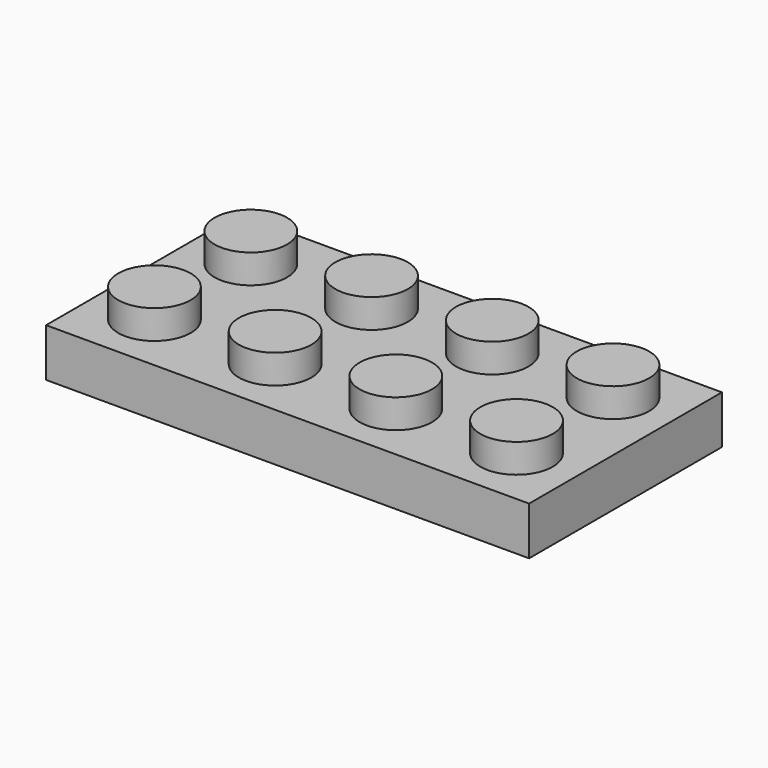
from build123d import *

# Parameters (mm, degrees)
F1_DEPTH = 3.175
F2_DEPTH = 5.08
F3_T     = -1.6002


# Not quite as in the source:
# - a feature names something its author has since deleted; it is built from what else it names


with BuildPart() as f1:
    # F0 (on Top) → F1 (new body)
    with BuildSketch(Plane.XY):
        with BuildLine():
            Line((-6.9955831819, 8.5962191019), (-38.8090831819, 8.5962191019))
            Line((-38.8090831819, 8.5962191019), (-38.8090831819, 4.6274691019))
            Line((-38.8090831819, 4.6274691019), (-37.2342831819, 4.6274691019))
            ThreePointArc((-37.2342831819, 4.6274691019), (-34.8466831819, 7.0150691019), (-32.4590831819, 4.6274691019))
            Line((-32.4590831819, 4.6274691019), (-29.2840831819, 4.6274691019))
            ThreePointArc((-29.2840831819, 4.6274691019), (-26.8964831819, 7.0150691019), (-24.5088831819, 4.6274691019))
            Line((-24.5088831819, 4.6274691019), (-21.3338831819, 4.6274691019))
            ThreePointArc((-21.3338831819, 4.6274691019), (-18.9462831819, 7.0150691019), (-16.5586831819, 4.6274691019))
            Line((-16.5586831819, 4.6274691019), (-13.3836831819, 4.6274691019))
            ThreePointArc((-13.3836831819, 4.6274691019), (-10.9960831819, 7.0150691019), (-8.6084831819, 4.6274691019))
            Line((-8.6084831819, 4.6274691019), (-6.9955831819, 4.6274691019))
            Line((-6.9955831819, 4.6274691019), (-6.9955831819, 8.5962191019))
        make_face()
        with BuildLine():
            Line((-37.2342831819, 4.6274691019), (-38.8090831819, 4.6274691019))
            Line((-38.8090831819, 4.6274691019), (-38.8090831819, 0.6587191019))
            Line((-38.8090831819, 0.6587191019), (-6.9955831819, 0.6587191019))
            Line((-6.9955831819, 0.6587191019), (-6.9955831819, 4.6274691019))
            Line((-6.9955831819, 4.6274691019), (-8.6084831819, 4.6274691019))
            ThreePointArc((-8.6084831819, 4.6274691019), (-10.9960831819, 2.2398691019), (-13.3836831819, 4.6274691019))
            Line((-13.3836831819, 4.6274691019), (-16.5586831819, 4.6274691019))
            ThreePointArc((-16.5586831819, 4.6274691019), (-18.9462831819, 2.2398691019), (-21.3338831819, 4.6274691019))
            Line((-21.3338831819, 4.6274691019), (-24.5088831819, 4.6274691019))
            ThreePointArc((-24.5088831819, 4.6274691019), (-26.8964831819, 2.2398691019), (-29.2840831819, 4.6274691019))
            Line((-29.2840831819, 4.6274691019), (-32.4590831819, 4.6274691019))
            ThreePointArc((-32.4590831819, 4.6274691019), (-34.8466831819, 2.2398691019), (-37.2342831819, 4.6274691019))
        make_face()
        with BuildLine():
            Line((-37.2342831819, -3.3100308981), (-38.8090831819, -3.3100308981))
            Line((-38.8090831819, -3.3100308981), (-38.8090831819, -7.2787808981))
            Line((-38.8090831819, -7.2787808981), (-6.9955831819, -7.2787808981))
            Line((-6.9955831819, -7.2787808981), (-6.9955831819, -3.3100308981))
            Line((-6.9955831819, -3.3100308981), (-8.6084831819, -3.3100308981))
            ThreePointArc((-8.6084831819, -3.3100308981), (-10.9960831819, -5.6976308981), (-13.3836831819, -3.3100308981))
            Line((-13.3836831819, -3.3100308981), (-16.5586831819, -3.3100308981))
            ThreePointArc((-16.5586831819, -3.3100308981), (-18.9462831819, -5.6976308981), (-21.3338831819, -3.3100308981))
            Line((-21.3338831819, -3.3100308981), (-24.5088831819, -3.3100308981))
            ThreePointArc((-24.5088831819, -3.3100308981), (-26.8964831819, -5.6976308981), (-29.2840831819, -3.3100308981))
            Line((-29.2840831819, -3.3100308981), (-32.4590831819, -3.3100308981))
            ThreePointArc((-32.4590831819, -3.3100308981), (-34.8466831819, -5.6976308981), (-37.2342831819, -3.3100308981))
        make_face()
        with BuildLine():
            Line((-6.9955831819, 0.6587191019), (-38.8090831819, 0.6587191019))
            Line((-38.8090831819, 0.6587191019), (-38.8090831819, -3.3100308981))
            Line((-38.8090831819, -3.3100308981), (-37.2342831819, -3.3100308981))
            ThreePointArc((-37.2342831819, -3.3100308981), (-34.8466831819, -0.9224308981), (-32.4590831819, -3.3100308981))
            Line((-32.4590831819, -3.3100308981), (-29.2840831819, -3.3100308981))
            ThreePointArc((-29.2840831819, -3.3100308981), (-26.8964831819, -0.9224308981), (-24.5088831819, -3.3100308981))
            Line((-24.5088831819, -3.3100308981), (-21.3338831819, -3.3100308981))
            ThreePointArc((-21.3338831819, -3.3100308981), (-18.9462831819, -0.9224308981), (-16.5586831819, -3.3100308981))
            Line((-16.5586831819, -3.3100308981), (-13.3836831819, -3.3100308981))
            ThreePointArc((-13.3836831819, -3.3100308981), (-10.9960831819, -0.9224308981), (-8.6084831819, -3.3100308981))
            Line((-8.6084831819, -3.3100308981), (-6.9955831819, -3.3100308981))
            Line((-6.9955831819, -3.3100308981), (-6.9955831819, 0.6587191019))
        make_face()
    extrude(amount=F1_DEPTH)

    # F0 (on Top) → F2 (join)
    with BuildSketch(Plane.XY):
        with BuildLine():
            Line((-32.4590831819, 4.6274691019), (-37.2342831819, 4.6274691019))
            ThreePointArc((-37.2342831819, 4.6274691019), (-34.8466831819, 2.2398691019), (-32.4590831819, 4.6274691019))
        make_face()
        with BuildLine():
            ThreePointArc((-32.4590831819, 4.6274691019), (-34.8466831819, 7.0150691019), (-37.2342831819, 4.6274691019))
            Line((-37.2342831819, 4.6274691019), (-32.4590831819, 4.6274691019))
        make_face()
        with BuildLine():
            ThreePointArc((-32.4590831819, -3.3100308981), (-34.8466831819, -0.9224308981), (-37.2342831819, -3.3100308981))
            Line((-37.2342831819, -3.3100308981), (-32.4590831819, -3.3100308981))
        make_face()
        with BuildLine():
            Line((-32.4590831819, -3.3100308981), (-37.2342831819, -3.3100308981))
            ThreePointArc((-37.2342831819, -3.3100308981), (-34.8466831819, -5.6976308981), (-32.4590831819, -3.3100308981))
        make_face()
        with BuildLine():
            Line((-24.5088831819, -3.3100308981), (-29.2840831819, -3.3100308981))
            ThreePointArc((-29.2840831819, -3.3100308981), (-26.8964831819, -5.6976308981), (-24.5088831819, -3.3100308981))
        make_face()
        with BuildLine():
            ThreePointArc((-24.5088831819, -3.3100308981), (-26.8964831819, -0.9224308981), (-29.2840831819, -3.3100308981))
            Line((-29.2840831819, -3.3100308981), (-24.5088831819, -3.3100308981))
        make_face()
        with BuildLine():
            Line((-24.5088831819, 4.6274691019), (-29.2840831819, 4.6274691019))
            ThreePointArc((-29.2840831819, 4.6274691019), (-26.8964831819, 2.2398691019), (-24.5088831819, 4.6274691019))
        make_face()
        with BuildLine():
            ThreePointArc((-24.5088831819, 4.6274691019), (-26.8964831819, 7.0150691019), (-29.2840831819, 4.6274691019))
            Line((-29.2840831819, 4.6274691019), (-24.5088831819, 4.6274691019))
        make_face()
        with BuildLine():
            ThreePointArc((-21.3338831819, -3.3100308981), (-18.9462831819, -5.6976308981), (-16.5586831819, -3.3100308981))
            Line((-16.5586831819, -3.3100308981), (-21.3338831819, -3.3100308981))
        make_face()
        with BuildLine():
            Line((-21.3338831819, -3.3100308981), (-16.5586831819, -3.3100308981))
            ThreePointArc((-16.5586831819, -3.3100308981), (-18.9462831819, -0.9224308981), (-21.3338831819, -3.3100308981))
        make_face()
        with BuildLine():
            Line((-21.3338831819, 4.6274691019), (-16.5586831819, 4.6274691019))
            ThreePointArc((-16.5586831819, 4.6274691019), (-18.9462831819, 7.0150691019), (-21.3338831819, 4.6274691019))
        make_face()
        with BuildLine():
            ThreePointArc((-21.3338831819, 4.6274691019), (-18.9462831819, 2.2398691019), (-16.5586831819, 4.6274691019))
            Line((-16.5586831819, 4.6274691019), (-21.3338831819, 4.6274691019))
        make_face()
        with BuildLine():
            Line((-13.3836831819, -3.3100308981), (-8.6084831819, -3.3100308981))
            ThreePointArc((-8.6084831819, -3.3100308981), (-10.9960831819, -0.9224308981), (-13.3836831819, -3.3100308981))
        make_face()
        with BuildLine():
            ThreePointArc((-13.3836831819, -3.3100308981), (-10.9960831819, -5.6976308981), (-8.6084831819, -3.3100308981))
            Line((-8.6084831819, -3.3100308981), (-13.3836831819, -3.3100308981))
        make_face()
        with BuildLine():
            ThreePointArc((-13.3836831819, 4.6274691019), (-10.9960831819, 2.2398691019), (-8.6084831819, 4.6274691019))
            Line((-8.6084831819, 4.6274691019), (-13.3836831819, 4.6274691019))
        make_face()
        with BuildLine():
            Line((-13.3836831819, 4.6274691019), (-8.6084831819, 4.6274691019))
            ThreePointArc((-8.6084831819, 4.6274691019), (-10.9960831819, 7.0150691019), (-13.3836831819, 4.6274691019))
        make_face()
    extrude(amount=F2_DEPTH)

    # F3
    f3_openings = [f1.faces().sort_by_distance(p)[0] for p in [
        (-22.902333, 0.658719, 0),
    ]]
    offset(amount=F3_T, openings=f3_openings, kind=Kind.INTERSECTION)


solid = f1.part
